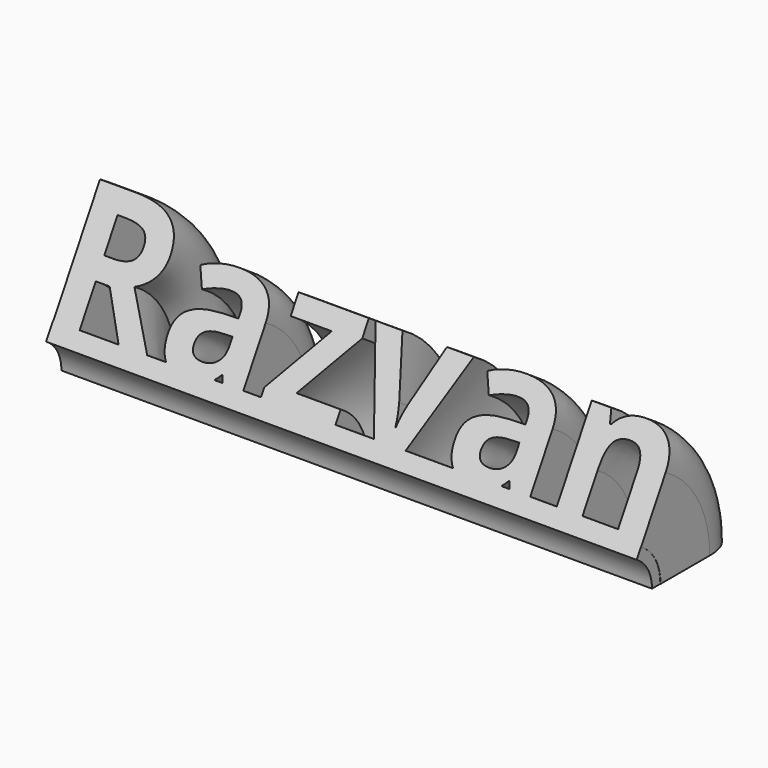
from build123d import *

# Parameters (mm, degrees)
F0_TEXT_SIZE = 40.1701868719
F1_W         = 137.3124
F1_H         = 4.054560326
F3_ANGLE     = 60


# Not quite as in the source:
# - Text() gives the source's letters only with a copy of the font that has no kerning and outlines rounded to 1/6400 em; it was checked with that copy


with BuildPart() as f3:
    # F0 (on Top) + F1 (on Top) → F3 (revolve)
    with BuildSketch(Plane.XY):
        with Locations((-76.1581659317, -11.014890857)):
            Text('Razvan', F0_TEXT_SIZE, font='Open Sans', font_style=FontStyle.BOLD, text_align=(TextAlign.LEFT, TextAlign.BOTTOM))
    with BuildSketch(Plane.XY):
        with Locations((-3.9859501802, -11.4203463309)):
            Rectangle(F1_W, F1_H)
    revolve(axis=Axis((0.3378801048, -22.3676599562, 0), (1, 0, 0)), revolution_arc=F3_ANGLE)


solid = f3.part
